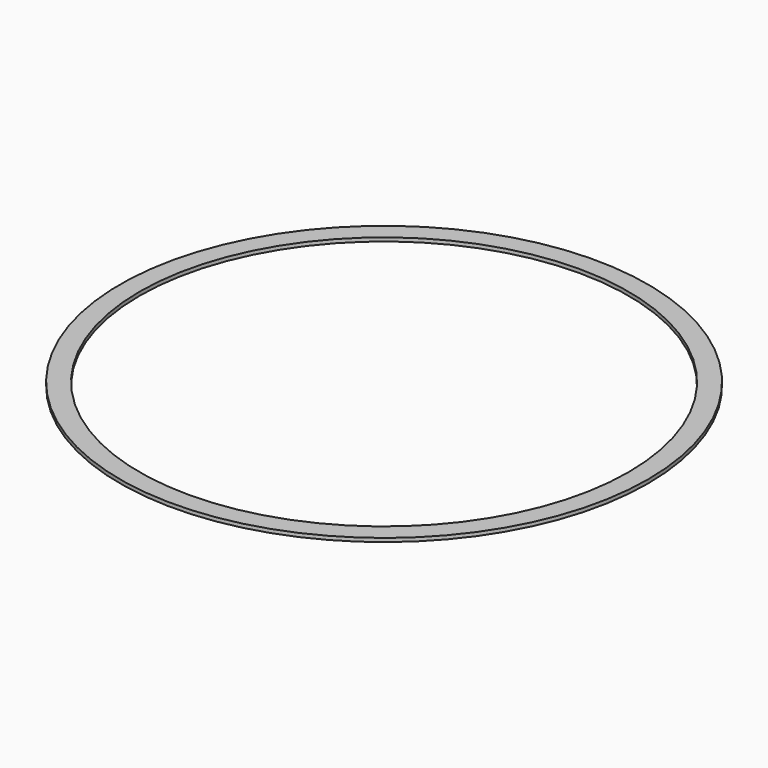
from build123d import *

# Parameters (mm, degrees)
F0_R     = 343.6493
F0_R_2   = 318.2493
F1_DEPTH = 4.7625


# Not quite as in the source:
# - a length typed as a fraction of an inch, garbled in the dataset ("3 / 203.2 mm" for 3/8 in), is restored


with BuildPart() as f1:
    # F0 (on Top) → F1 (new body)
    with BuildSketch(Plane.XY):
        Circle(F0_R)
        Circle(F0_R_2, mode=Mode.SUBTRACT)
    extrude(amount=F1_DEPTH)


solid = f1.part
